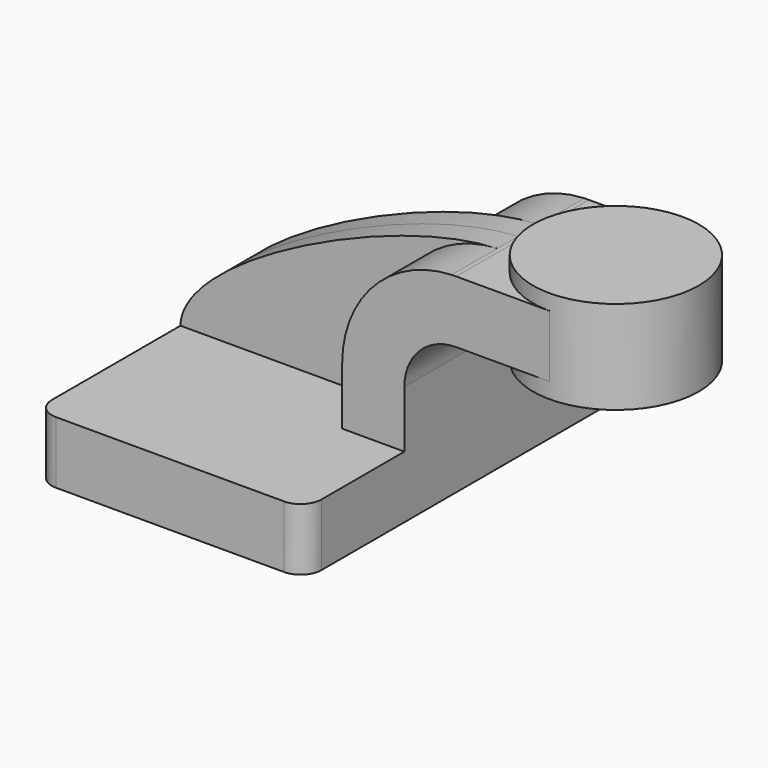
from build123d import *

# Parameters (mm, degrees)
F1_DEPTH = 63.5
F0_W     = 25.4
F0_H     = 19.05
F2_DEPTH = 25.4
F3_DEPTH = 7.9375
F5_R     = 6.35


# Not quite as in the source:
# - a feature names something its author has since deleted; it is built from what else it names


with BuildPart() as f1:
    # F0 (on Front) → F1 (new body, symmetric)
    with BuildSketch(Plane.XZ):
        Polygon((22.225, 9.525), (-41.275, 9.525), (-41.275, -9.525), (41.275, -9.525), (41.275, 9.525), align=None)
    extrude(amount=F1_DEPTH, both=True)

    # F0 (on Front) → F2 (join, symmetric)
    with BuildSketch(Plane.XZ):
        with BuildLine():
            Line((22.225, 26.9875), (22.225, 9.525))
            Line((22.225, 9.525), (41.275, 9.525))
            Line((41.275, 9.525), (41.275, 26.9875))
            ThreePointArc((41.275, 26.9875), (45.9246798487, 38.2128201513), (57.15, 42.8625))
            Line((57.15, 42.8625), (60.325, 42.8625))
            Line((60.325, 42.8625), (60.325, 61.9125))
            Line((60.325, 61.9125), (57.15, 61.9125))
            add(Edge.make_bspline(
                [(55.7518836795, 61.8845041086), (56.2255175188, 61.9006022789), (56.6916659887, 61.909979921), (57.15, 61.9125)],
                knots=[109.8544384291, 109.8544384291, 109.8544384291, 109.8544384291, 111.4985685166, 111.4985685166, 111.4985685166, 111.4985685166], degree=3))
            ThreePointArc((55.7518836795, 61.8845041086), (31.9648373293, 51.1838469609), (22.225, 26.9875))
        make_face()
        with Locations((73.025, 52.3875)):
            Rectangle(F0_W, F0_H)
    extrude(amount=F2_DEPTH, both=True)

    # F0 (on Front) → F3 (join, symmetric)
    with BuildSketch(Plane.XZ):
        with BuildLine():
            add(Edge.make_bspline(
                [(-41.275, 9.525), (-40.9585584382, 29.7301590249), (24.1054952085, 60.8088863876), (55.7518836795, 61.8845041086)],
                knots=[0, 0, 0, 0, 109.8544384291, 109.8544384291, 109.8544384291, 109.8544384291], degree=3))
            Line((-41.275, 9.525), (22.225, 9.525))
            Line((22.225, 9.525), (22.225, 26.9875))
            ThreePointArc((22.225, 26.9875), (31.9648373293, 51.1838469609), (55.7518836795, 61.8845041086))
        make_face()
    extrude(amount=F3_DEPTH, both=True)

    # F5
    f5_edges = [f1.edges().sort_by_distance(p)[0] for p in [
        (41.275, -63.5, 0),
        (-41.275, -63.5, 0),
        (41.275, 63.5, 0),
        (-41.275, 63.5, 0),
    ]]
    fillet(f5_edges, radius=F5_R)


with BuildPart() as f4:
    # F0 (on Front) → F4 (revolve)
    with BuildSketch(Plane.XZ):
        Polygon((85.725, 66.675), (85.725, 61.9125), (85.725, 42.8625), (85.725, 38.1), (111.125, 38.1), (111.125, 66.675), align=None)
    revolve(axis=Axis((85.725, 0, 52.3875), (0, 0, -1)))


solid = Compound([f1.part, f4.part])
